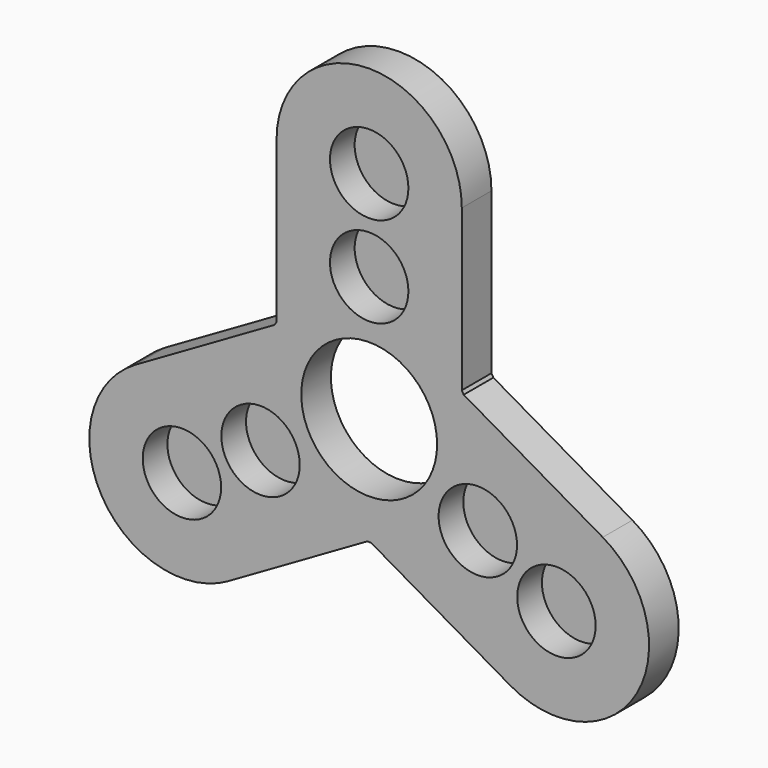
from build123d import *

# Parameters (mm, degrees)
F0_R     = 6.35
F0_R_2   = 11
F1_DEPTH = 6
F2_DEPTH = 1


# Not quite as in the source:
# - a feature names something its author has since deleted; it is built from what else it names


with BuildPart() as f1:
    # F0 (on Front) → F1 (new body)
    with BuildSketch(Plane.XZ):
        with BuildLine():
            Line((-22.8229079964, -30.4973201511), (-0.306247498, -17.4973201511))
            ThreePointArc((-0.306247498, -17.4973201511), (0, -17.5), (0.306247498, -17.4973201511))
            Line((0.306247498, -17.4973201511), (22.8229079964, -30.4973201511))
            ThreePointArc((22.8229079964, -30.4973201511), (43.3132890532, -25.0069390943), (37.8229079964, -4.5165580376))
            Line((37.8229079964, -4.5165580376), (15.306247498, 8.4834419624))
            ThreePointArc((15.306247498, 8.4834419624), (15.1554445662, 8.75), (15, 9.0138781887))
            Line((15, 9.0138781887), (15, 35.0138781887))
            ThreePointArc((15, 35.0138781887), (0, 50.0138781887), (-15, 35.0138781887))
            Line((-15, 35.0138781887), (-15, 9.0138781887))
            ThreePointArc((-15, 9.0138781887), (-15.1554445662, 8.75), (-15.306247498, 8.4834419624))
            Line((-15.306247498, 8.4834419624), (-37.8229079964, -4.5165580376))
            ThreePointArc((-37.8229079964, -4.5165580376), (-43.3132890532, -25.0069390943), (-22.8229079964, -30.4973201511))
        make_face()
        with Locations((-30.3229079964, -17.5069390943)):
            Circle(F0_R, mode=Mode.SUBTRACT)
        with Locations((-17.5923345608, -10.1569390943)):
            Circle(F0_R, mode=Mode.SUBTRACT)
        with Locations((30.3229079964, -17.5069390943)):
            Circle(F0_R, mode=Mode.SUBTRACT)
        with Locations((17.5923345608, -10.1569390943)):
            Circle(F0_R, mode=Mode.SUBTRACT)
        Circle(F0_R_2, mode=Mode.SUBTRACT)
        with Locations((0, 20.3138781887)):
            Circle(F0_R, mode=Mode.SUBTRACT)
        with Locations((0, 35.0138781887)):
            Circle(F0_R, mode=Mode.SUBTRACT)
    extrude(amount=F1_DEPTH)

    # F0 (on Front) → F2 (join)
    with BuildSketch(Plane.XZ):
        with Locations((-30.3229079964, -17.5069390943)):
            Circle(F0_R)
        with Locations((-17.5923345608, -10.1569390943)):
            Circle(F0_R)
        with Locations((17.5923345608, -10.1569390943)):
            Circle(F0_R)
        with Locations((30.3229079964, -17.5069390943)):
            Circle(F0_R)
        with Locations((0, 20.3138781887)):
            Circle(F0_R)
        with Locations((0, 35.0138781887)):
            Circle(F0_R)
    extrude(amount=F2_DEPTH)


solid = f1.part
